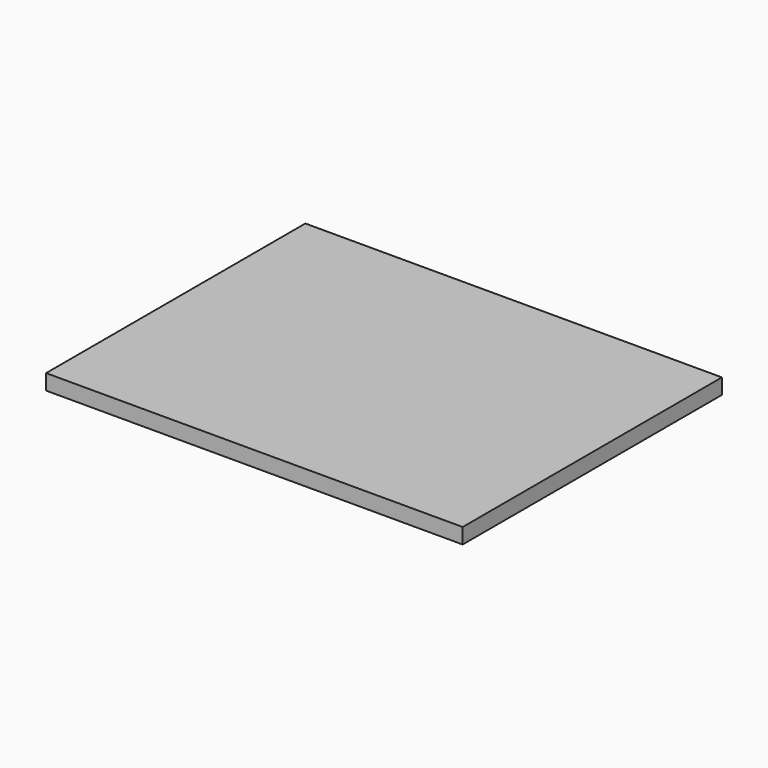
from build123d import *

# Parameters (mm, degrees)
F0_W     = 270
F0_H     = 210
F1_DEPTH = 10


# Not quite as in the source:
# - a feature names something its author has since deleted; it is built from what else it names


with BuildPart() as f1:
    # F0 (on Top) → F1 (new body)
    with BuildSketch(Plane.XY):
        Rectangle(F0_W, F0_H)
    extrude(amount=F1_DEPTH)


solid = f1.part
